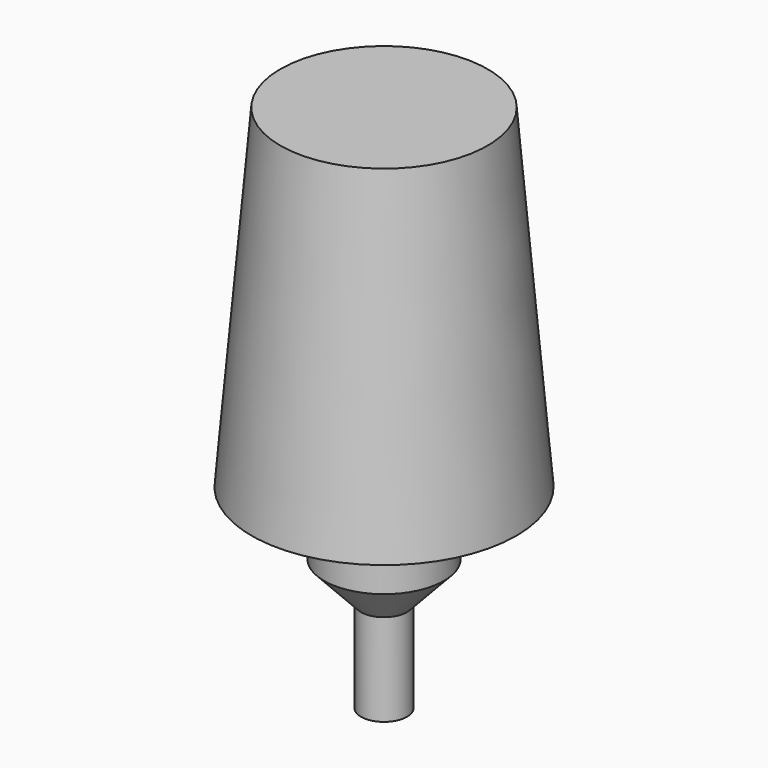
from build123d import *


# Not quite as in the source:
# - a fillet or chamfer that OpenCascade refuses, or shapes differently, is made with other operations: its cross-section is extruded or revolved along the edge and cut away or added


with BuildPart() as f1:
    # F0 (on Front) → F1 (revolve)
    with BuildSketch(Plane.XZ):
        Polygon((0, -16.9278544536), (0, 0), (0, 29), (-9, 29), (-11.5, 0), (-4, 0), (-4, -2.5), (-5.2, -2.5), (-5.2, -5.5), (-2, -8.9278544536), (-2, -16.9278544536), align=None)
    revolve(axis=Axis((0, 0, 14.5), (0, 0, 1)))

    # F2: fillet of radius 3 on 1 edges, made by hand

    # F2_s1 → F2_t2 (revolve)
    with BuildSketch(Plane.XZ):
        with BuildLine():
            ThreePointArc((-4, -0.1), (-4.316718427, -1.4416407865), (-5.2, -2.5))
            Line((-5.2, -2.5), (-5.164, -2.548))
            ThreePointArc((-5.164, -2.548), (-4.6, -2.56), (-4, -2.56))
            Line((-4, -2.56), (-3.94, -2.5))
            Line((-3.94, -2.5), (-3.94, -0.1))
            Line((-3.94, -0.1), (-4, -0.1))
        make_face()
    revolve(axis=Axis((0, 0, -2.5), (0, 0, 1)))


solid = f1.part
